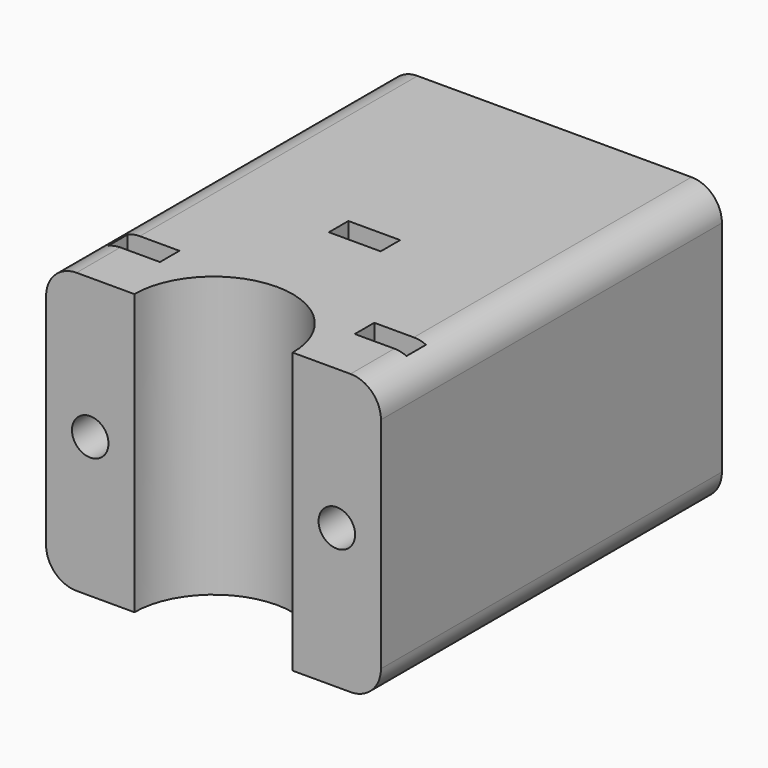
from build123d import *

# Parameters (mm, degrees)
F0_W         = 55
F0_H         = 46
F5_DEPTH     = 70
F1_W         = 7.25
F1_H         = 70
F6_DEPTH     = 23
F7_D         = 6
F7_DEPTH     = 15
F7_TIP       = 1.8025818571
F9_DEPTH     = 4
F10_W        = 36
F10_H        = 36
F11_DEPTH    = 4
F12_D        = 6
F12_DEPTH    = 38
F12_TIP      = 1.8025818571
F14_DEPTH    = 4
F15_T1_DEPTH = 95
F16_DEPTH    = 33
F17_DEPTH    = 10


# Not quite as in the source:
# - a fillet or chamfer that OpenCascade refuses, or shapes differently, is made with other operations: its cross-section is extruded or revolved along the edge and cut away or added


with BuildPart() as f5:
    # F0 (on Front) → F5 (new body)
    with BuildSketch(Plane.XZ):
        Rectangle(F0_W, F0_H)
    extrude(amount=-F5_DEPTH)

    # F1 (on Top) → F6 (intersect, symmetric)
    with BuildSketch(Plane.XY):
        with BuildLine():
            Line((-20.25, 0), (-13, 0))
            ThreePointArc((-13, 0), (0, 13), (13, 0))
            Line((13, 0), (20.25, 0))
            Line((20.25, 0), (20.25, 70))
            Line((20.25, 70), (-20.25, 70))
            Line((-20.25, 70), (-20.25, 0))
        make_face()
        with Locations((-23.875, 35)):
            Rectangle(F1_W, F1_H)
        with Locations((23.875, 35)):
            Rectangle(F1_W, F1_H)
    extrude(amount=F6_DEPTH, both=True, mode=Mode.INTERSECT)

    # F7
    with Locations(Plane.XZ):
        with Locations((-20.25, 0), (20.25, 0)):
            Hole(F7_D / 2, depth=F7_DEPTH)
            with Locations((0, 0, -(F7_DEPTH + F7_TIP / 2))):  # 118° drill point
                Cone(0, F7_D / 2, F7_TIP, mode=Mode.SUBTRACT)

    # F8 (on offset) → F9 (cut)
    with BuildSketch(Plane.XZ.offset(-9)):
        Polygon((-24.5, 2.4537386441), (-24.5, 2.25), (-24.5, -2.4537386441), (-20.25, -4.9074772881), (-16, -2.4537386441), (-16, 2), (-16, 2.4537386441), (-20.25, 4.9074772881), align=None)
        Polygon((-24.5, 23), (-24.5, 2.4537386441), (-20.25, 4.9074772881), (-16, 2.4537386441), (-16, 23), align=None)
        Polygon((24.5, 2.4537386441), (24.5, 23), (16, 23), (16, 2.4537386441), (16, 2), (16, -2.4537386441), (20.25, -4.9074772881), (24.5, -2.4537386441), (24.5, 2.25), align=None)
    extrude(amount=-F9_DEPTH, mode=Mode.SUBTRACT)

    # F10 (on offset) → F11 (cut)
    with BuildSketch(Plane.XZ.offset(-66)):
        Rectangle(F10_W, F10_H)
    extrude(amount=-F11_DEPTH, mode=Mode.SUBTRACT)

    # F12
    with Locations(Plane(origin=(0, 66, 0), x_dir=(1, 0, 0), z_dir=(0, 1, 0))):
        with Locations((0, 0)):
            Hole(F12_D / 2, depth=F12_DEPTH)
            with Locations((0, 0, -(F12_DEPTH + F12_TIP / 2))):  # 118° drill point
                Cone(0, F12_D / 2, F12_TIP, mode=Mode.SUBTRACT)

    # F13 (on offset) → F14 (cut)
    with BuildSketch(Plane.XZ.offset(-29)):
        Polygon((-4.25, 2.4537386441), (-4.25, 2.25), (-4.25, -2.4537386441), (0, -4.9074772881), (4.25, -2.4537386441), (4.25, 2.0686155439), (4.25, 2.4537386441), (0, 4.9074772881), align=None)
        Polygon((-4.25, 23), (-4.25, 2.4537386441), (0, 4.9074772881), (4.25, 2.4537386441), (4.25, 23), align=None)
        with BuildLine():
            ThreePointArc((23.5, 14), (22.0355339059, 17.5355339059), (18.5, 19))
            Line((18.5, 19), (13.25, 19))
            ThreePointArc((13.25, 19), (9.7144660941, 17.5355339059), (8.25, 14))
            Line((8.25, 14), (8.25, -14))
            ThreePointArc((8.25, -14), (9.7144660941, -17.5355339059), (13.25, -19))
            Line((13.25, -19), (18.5, -19))
            ThreePointArc((18.5, -19), (22.0355339059, -17.5355339059), (23.5, -14))
            Line((23.5, -14), (23.5, 14))
        make_face()
        with BuildLine():
            Line((-13.25, 19), (-18.5, 19))
            ThreePointArc((-18.5, 19), (-22.0355339059, 17.5355339059), (-23.5, 14))
            Line((-23.5, 14), (-23.5, -14))
            ThreePointArc((-23.5, -14), (-22.0355339059, -17.5355339059), (-18.5, -19))
            Line((-18.5, -19), (-13.25, -19))
            ThreePointArc((-13.25, -19), (-9.7144660941, -17.5355339059), (-8.25, -14))
            Line((-8.25, -14), (-8.25, 14))
            ThreePointArc((-8.25, 14), (-9.7144660941, 17.5355339059), (-13.25, 19))
        make_face()
    extrude(amount=-F14_DEPTH, mode=Mode.SUBTRACT)

    # F15: fillet of radius 5 on 4 edges, made by hand

    # F15_s2 → F15_t1 (cut)
    with BuildSketch(Plane.XZ.offset(-82.5)):
        with BuildLine():
            ThreePointArc((-22.5, 23), (-26.0355339059, 21.5355339059), (-27.5, 18))
            Line((-27.5, 18), (-27.5, 23))
            Line((-27.5, 23), (-22.5, 23))
        make_face()
        with BuildLine():
            ThreePointArc((22.5, 23), (26.0355339059, 21.5355339059), (27.5, 18))
            Line((27.5, 18), (27.5, 23))
            Line((27.5, 23), (22.5, 23))
        make_face()
        with BuildLine():
            ThreePointArc((-22.5, -23), (-26.0355339059, -21.5355339059), (-27.5, -18))
            Line((-27.5, -18), (-27.5, -23))
            Line((-27.5, -23), (-22.5, -23))
        make_face()
        with BuildLine():
            ThreePointArc((22.5, -23), (26.0355339059, -21.5355339059), (27.5, -18))
            Line((27.5, -18), (27.5, -23))
            Line((27.5, -23), (22.5, -23))
        make_face()
    extrude(amount=F15_T1_DEPTH, mode=Mode.SUBTRACT)

    # F13 (on offset) → F16 (cut)
    with BuildSketch(Plane.XZ.offset(-29)):
        with BuildLine():
            ThreePointArc((23.5, 14), (22.0355339059, 17.5355339059), (18.5, 19))
            Line((18.5, 19), (13.25, 19))
            ThreePointArc((13.25, 19), (9.7144660941, 17.5355339059), (8.25, 14))
            Line((8.25, 14), (8.25, -14))
            ThreePointArc((8.25, -14), (9.7144660941, -17.5355339059), (13.25, -19))
            Line((13.25, -19), (18.5, -19))
            ThreePointArc((18.5, -19), (22.0355339059, -17.5355339059), (23.5, -14))
            Line((23.5, -14), (23.5, 14))
        make_face()
        with BuildLine():
            Line((-13.25, 19), (-18.5, 19))
            ThreePointArc((-18.5, 19), (-22.0355339059, 17.5355339059), (-23.5, 14))
            Line((-23.5, 14), (-23.5, -14))
            ThreePointArc((-23.5, -14), (-22.0355339059, -17.5355339059), (-18.5, -19))
            Line((-18.5, -19), (-13.25, -19))
            ThreePointArc((-13.25, -19), (-9.7144660941, -17.5355339059), (-8.25, -14))
            Line((-8.25, -14), (-8.25, 14))
            ThreePointArc((-8.25, 14), (-9.7144660941, 17.5355339059), (-13.25, 19))
        make_face()
    extrude(amount=-F16_DEPTH, mode=Mode.SUBTRACT)

    # F13 (on offset) → F17 (cut)
    with BuildSketch(Plane.XZ.offset(-29)):
        with BuildLine():
            ThreePointArc((23.5, 14), (22.0355339059, 17.5355339059), (18.5, 19))
            Line((18.5, 19), (13.25, 19))
            ThreePointArc((13.25, 19), (9.7144660941, 17.5355339059), (8.25, 14))
            Line((8.25, 14), (8.25, -14))
            ThreePointArc((8.25, -14), (9.7144660941, -17.5355339059), (13.25, -19))
            Line((13.25, -19), (18.5, -19))
            ThreePointArc((18.5, -19), (22.0355339059, -17.5355339059), (23.5, -14))
            Line((23.5, -14), (23.5, 14))
        make_face()
        with BuildLine():
            Line((-13.25, 19), (-18.5, 19))
            ThreePointArc((-18.5, 19), (-22.0355339059, 17.5355339059), (-23.5, 14))
            Line((-23.5, 14), (-23.5, -14))
            ThreePointArc((-23.5, -14), (-22.0355339059, -17.5355339059), (-18.5, -19))
            Line((-18.5, -19), (-13.25, -19))
            ThreePointArc((-13.25, -19), (-9.7144660941, -17.5355339059), (-8.25, -14))
            Line((-8.25, -14), (-8.25, 14))
            ThreePointArc((-8.25, 14), (-9.7144660941, 17.5355339059), (-13.25, 19))
        make_face()
    extrude(amount=F17_DEPTH, mode=Mode.SUBTRACT)


solid = f5.part
